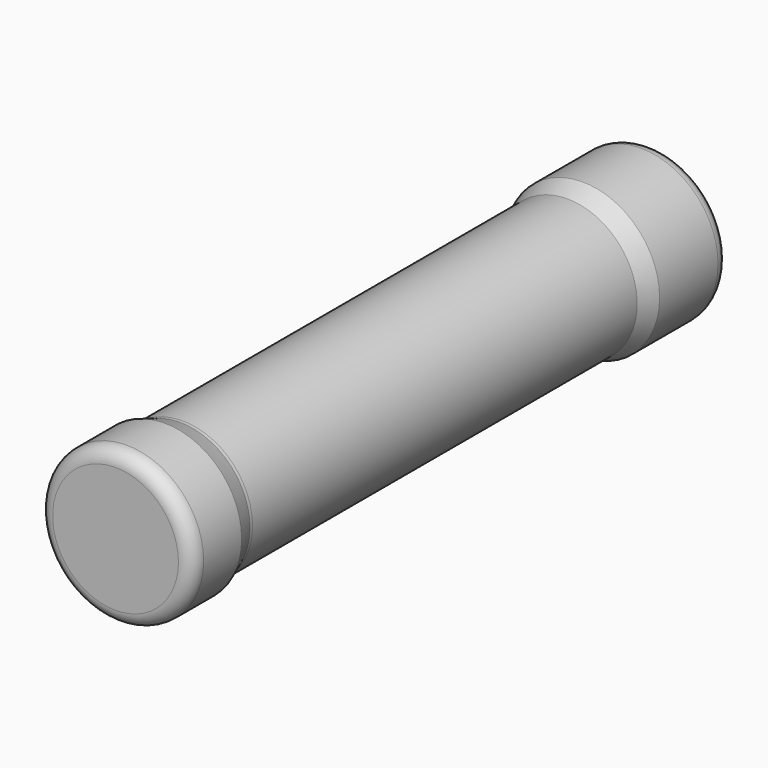
from build123d import *

# Parameters (mm, degrees)
F0_R          = 34.925
F0_R_2        = 28.575
F1_DEPTH      = 304.8
F2_R          = 34.925
F3_DEPTH      = 6.35
F4_R          = 34.925
F5_DEPTH      = 6.35
F6_R          = 6.35
F7_R          = 6.35
F8_W          = 228.6
F8_H          = 3.175
F10_S5_R      = 34.925
F10_T6_DEPTH  = 52
F10_S11_R     = 31.75
F10_T12_DEPTH = 51
F11_R         = 6.35
F12_DEPTH     = 25.4


# Not quite as in the source:
# - a fillet or chamfer that OpenCascade refuses, or shapes differently, is made with other operations: its cross-section is extruded or revolved along the edge and cut away or added


with BuildPart() as f1:
    # F0 (on Front) → F1 (new body)
    with BuildSketch(Plane.XZ):
        Circle(F0_R)
        Circle(F0_R_2, mode=Mode.SUBTRACT)
    extrude(amount=F1_DEPTH)

    # F2 (on face) → F3 (join)
    with BuildSketch(Plane.XZ.offset(304.8)):
        Circle(F2_R)
    extrude(amount=-F3_DEPTH)

    # F4 (on face) → F5 (join)
    with BuildSketch(Plane(origin=(0, 0, 0), x_dir=(-1, 0, 0), z_dir=(0, 1, 0))):
        Circle(F4_R)
    extrude(amount=-F5_DEPTH)

    # F6
    f6_edges = [f1.edges().sort_by_distance(p)[0] for p in [
        (-34.925, 0, 0),
    ]]
    fillet(f6_edges, radius=F6_R)

    # F7
    f7_edges = [f1.edges().sort_by_distance(p)[0] for p in [
        (-34.925, -304.8, 0),
    ]]
    fillet(f7_edges, radius=F7_R)

    # F8 (on Right) → F9 (revolve, cut)
    with BuildSketch(Plane.YZ):
        with Locations((-152.4, -33.3375)):
            Rectangle(F8_W, F8_H)
    revolve(axis=Axis((0, -304.8, 0), (0, -1, 0)), mode=Mode.SUBTRACT)

    # F10: chamfer of 10.16 x 3.6979375801 on 2 edges, made by hand


with BuildPart() as f10_tool2:
    # F10_s3 → F10_t4 (revolve)
    with BuildSketch(Plane.YZ):
        Polygon((-48.26, -31.75), (-38.1, -35.4479375801), (-38.1, -31.75), align=None)
    revolve(axis=Axis((0, -38.1, 0), (0, -1, 0)))

    # F10_s5 → F10_t6 (intersect, symmetric)
    with BuildSketch(Plane.XZ.offset(43.2)):
        Circle(F10_S5_R)
    extrude(amount=F10_T6_DEPTH, both=True, mode=Mode.INTERSECT)


with BuildPart() as f1_1:
    add(f1.part)

    # F10_t1: union F10_tool2
    add(f10_tool2.part)


with BuildPart() as f10_tool8:
    # F10_s9 → F10_t10 (revolve)
    with BuildSketch(Plane.XY):
        Polygon((34.925, -276.86), (31.2270624199, -266.7), (34.925, -266.7), align=None)
    revolve(axis=Axis((0, -266.7, 0), (0, -1, 0)))

    # F10_s11 → F10_t12 (cut, symmetric)
    with BuildSketch(Plane.XZ.offset(271.8)):
        Circle(F10_S11_R)
    extrude(amount=F10_T12_DEPTH, both=True, mode=Mode.SUBTRACT)


with BuildPart() as f1_2:
    add(f1_1.part)

    # F10_t7: cut F10_tool8
    add(f10_tool8.part, mode=Mode.SUBTRACT)

    # F11 (on face) → F12 (cut)
    with BuildSketch(Plane(origin=(0, 0, 0), x_dir=(-1, 0, 0), z_dir=(0, 1, 0))):
        Circle(F11_R)
    extrude(amount=-F12_DEPTH, mode=Mode.SUBTRACT)


solid = f1_2.part
